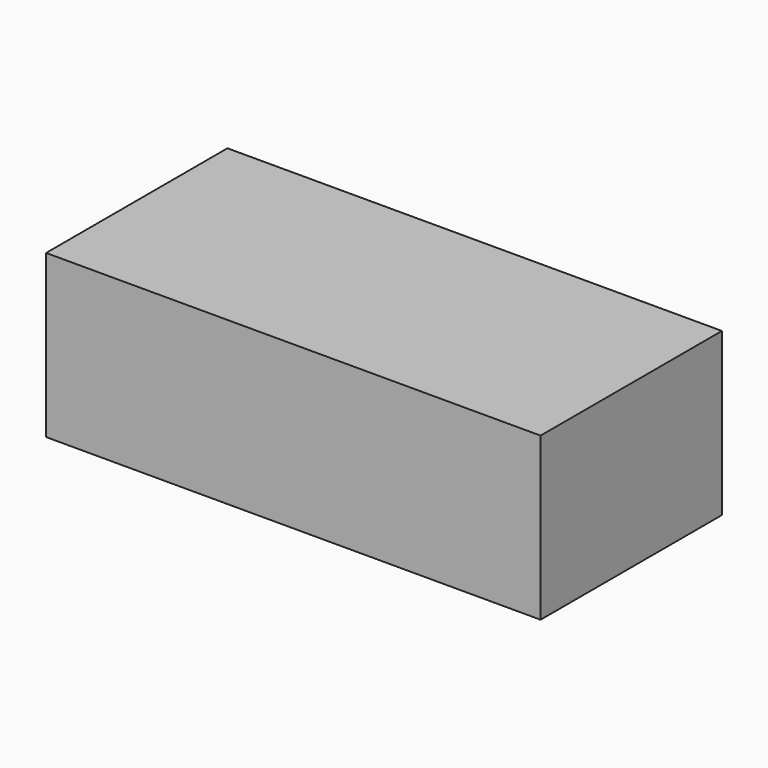
from build123d import *

# Parameters (mm, degrees)
F0_W     = 112.3474985361
F0_H     = 51.5004433692
F1_DEPTH = 18.415


# Not quite as in the source:
# - the program builds the solid bodies; features that only make, move or delete a surface that nothing else refers to are left out


with BuildPart() as f1:
    # F0 (on Top) → F1 (new body, symmetric)
    with BuildSketch(Plane.XY):
        Rectangle(F0_W, F0_H)
    extrude(amount=F1_DEPTH, both=True)


solid = f1.part
